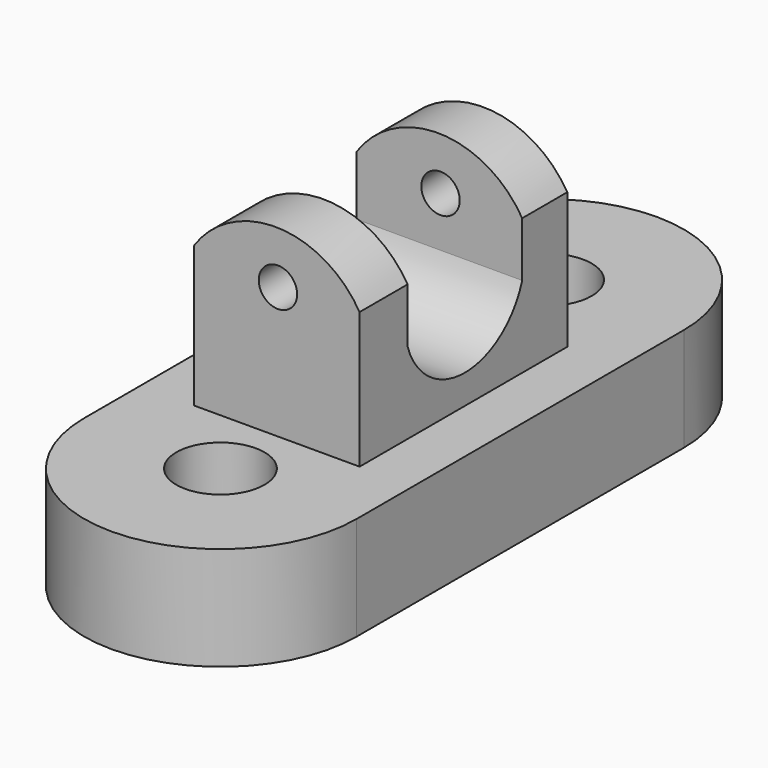
from build123d import *

# Parameters (mm, degrees)
F0_R      = 8.2136813159
F0_R_2    = 8.2169
F1_DEPTH  = 19.304
F2_W      = 42.0680484259
F2_H      = 48.3717918396
F3_DEPTH  = 34.29
F4_DEPTH  = 5.588
F5_DEPTH  = 5.588
F8_DEPTH  = 34.29
F9_DEPTH  = 60.198
F10_R     = 3.577492803
F11_DEPTH = 65.786


# Not quite as in the source:
# - a feature names something its author has since deleted; it is built from what else it names


with BuildPart() as f1:
    # F0 (on Top) → F1 (new body)
    with BuildSketch(Plane.XY):
        with BuildLine():
            Line((25.4, -38.1), (25.4, 38.1))
            ThreePointArc((25.4, 38.1), (0, 12.7), (-25.4, 38.1))
            Line((-25.4, 38.1), (-25.4, -38.1))
            ThreePointArc((-25.4, -38.1), (0, -12.7), (25.4, -38.1))
        make_face()
        with BuildLine():
            ThreePointArc((-25.4, -38.1), (0, -63.5), (25.4, -38.1))
            ThreePointArc((25.4, -38.1), (0, -12.7), (-25.4, -38.1))
        make_face()
        with Locations((0, -38.1)):
            Circle(F0_R, mode=Mode.SUBTRACT)
        with BuildLine():
            ThreePointArc((-25.4, 38.1), (0, 12.7), (25.4, 38.1))
            ThreePointArc((25.4, 38.1), (0, 63.5), (-25.4, 38.1))
        make_face()
        with Locations((0, 38.1)):
            Circle(F0_R_2, mode=Mode.SUBTRACT)
    extrude(amount=F1_DEPTH)

    # F2 (on face) → F3 (join)
    with BuildSketch(Plane.XY.offset(19.304)):
        with Locations((-0.0028242129, -0.8024219424)):
            Rectangle(F2_W, F2_H)
    extrude(amount=F3_DEPTH)

    # F4 (cut): a face of the model
    f4_faces = [f1.faces().sort_by_distance(p)[0] for p in [
        (21.0312, -0.8024219424, 36.449),
    ]]
    extrude(f4_faces, amount=-F4_DEPTH, mode=Mode.SUBTRACT)

    # F5 (cut): a face of the model
    f5_faces = [f1.faces().sort_by_distance(p)[0] for p in [
        (-21.0368484259, -0.8024219424, 36.449),
    ]]
    extrude(f5_faces, amount=-F5_DEPTH, mode=Mode.SUBTRACT)

    # F7 (on face) → F8 (cut)
    with BuildSketch(Plane.YZ.offset(15.4432)):
        with BuildLine():
            Line((12.8851897717, 53.594), (-13.8123355974, 53.594))
            Line((-13.8123355974, 53.594), (-13.8123355974, 34.4488508999))
            ThreePointArc((-13.8123355974, 34.4488508999), (-0.4635729128, 24.7413409198), (12.8851897717, 34.4488508999))
            Line((12.8851897717, 34.4488508999), (12.8851897717, 53.594))
        make_face()
    extrude(amount=-F8_DEPTH, mode=Mode.SUBTRACT)

    # F6 (on face) → F9 (cut)
    with BuildSketch(Plane.XZ.offset(24.9883178622)):
        with BuildLine():
            ThreePointArc((-15.4488484259, 45.4977191985), (0.2250638301, 53.5401239092), (15.4432, 44.6654334664))
            Line((15.4432, 44.6654334664), (15.4432, 53.594))
            Line((15.4432, 53.594), (-15.4488484259, 53.594))
            Line((-15.4488484259, 53.594), (-15.4488484259, 45.4977191985))
        make_face()
    extrude(amount=-F9_DEPTH, mode=Mode.SUBTRACT)

    # F10 (on face) → F11 (cut)
    with BuildSketch(Plane.XZ.offset(24.9883178622)):
        with Locations((0.2250638301, 43.7909998)):
            Circle(F10_R)
    extrude(amount=-F11_DEPTH, mode=Mode.SUBTRACT)


solid = f1.part
